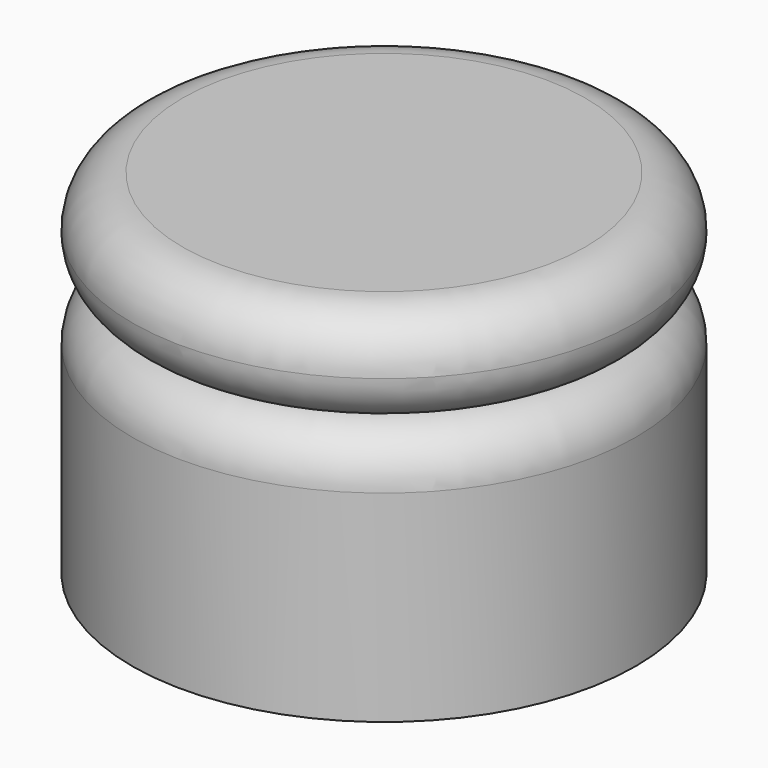
from build123d import *

# Parameters (mm, degrees)
F2_R = 2.53999


# Not quite as in the source:
# - a fillet or chamfer is up to 0.001 mm smaller than in the source, because OpenCascade refuses the exact size


with BuildPart() as f1:
    # F0 (on Front) → F1 (revolve)
    with BuildSketch(Plane.XZ):
        with BuildLine():
            Line((0, 17.78), (0, 0))
            Line((0, 0), (12.7, 0))
            Line((12.7, 0), (12.7, 10.16))
            ThreePointArc((12.7, 10.16), (11.9560512242, 11.9560512242), (10.16, 12.7))
            ThreePointArc((10.16, 12.7), (11.9560512242, 13.4439487758), (12.7, 15.24))
            Line((12.7, 15.24), (12.7, 17.78))
            Line((12.7, 17.78), (0, 17.78))
        make_face()
    revolve(axis=Axis((0, 0, 8.89), (0, 0, -1)))

    # F2 (radius 2.54 in the source; OpenCascade refuses exactly that, so slightly less here)
    f2_edges = [f1.edges().sort_by_distance(p)[0] for p in [
        (-12.7, 0, 17.78),
    ]]
    fillet(f2_edges, radius=F2_R)


solid = f1.part
